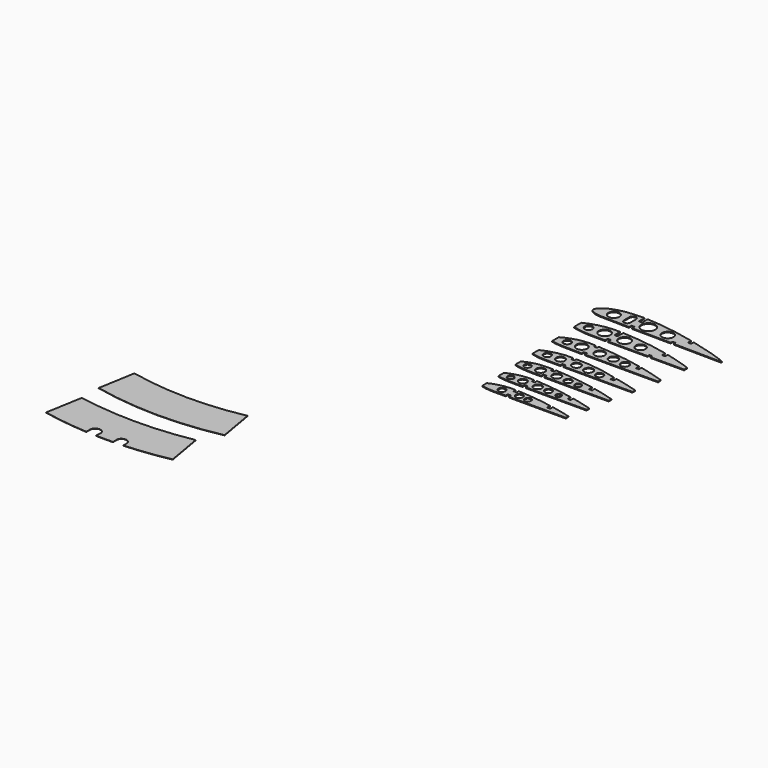
from build123d import *

# Parameters (mm, degrees)
F0_R     = 11.0622151746
F0_R_2   = 13.8024255372
F0_R_3   = 11.3624106866
F1_DEPTH = 1.5875
F0_R_4   = 7.8101063495
F0_R_5   = 11.4767284211
F0_R_6   = 11.8200632114
F0_R_7   = 9.8314713696
F0_R_8   = 7.5345089111
F0_R_9   = 10.9529535392
F0_R_10  = 10.0879453798
F0_R_11  = 8.94065382
F0_R_12  = 8.1637602934
F0_R_13  = 7.4256431867
F0_R_14  = 8.671057932
F0_R_15  = 8.7945693521
F0_R_16  = 8.7340618452
F0_R_17  = 7.4133759763
F0_R_18  = 6.6977708364
F0_R_19  = 8.7178990493
F0_R_20  = 8.6654991063
F0_R_21  = 7.401165003
F0_R_22  = 6.2678513164
F0_R_23  = 6.2709150441
F0_R_24  = 7.8954222452
F0_R_25  = 8.25631298
F0_R_26  = 7.1918059299
F0_R_27  = 5.3987930497
F0_R_28  = 7.1117244514
F0_R_29  = 7.1354689901
F0_R_30  = 6.3367708827
F3_DEPTH = 0.6


# Not quite as in the source:
# - a length typed as a fraction of an inch, garbled in the dataset ("3 / 203.2 mm" for 3/8 in), is restored


with BuildPart() as f1:
    # F0 (on Top) → F1 (new body)
    with BuildSketch(Plane.XY):
        with BuildLine():
            add(Edge.make_bspline(
                [(1167.916059494, 673.0018258095), (1177.8327603734, 680.2652288209), (1199.7700553684, 687.2151988613), (1229.9858664166, 688.5294701263), (1239.9305907432, 688.4111456973)],
                knots=[0, 0, 0, 0, 0.1072430775, 0.1545371155, 0.1545371155, 0.1545371155, 0.1545371155], degree=3))
            add(Edge.make_bspline(
                [(1239.9305907431, 649.5218357149), (1234.8037192798, 649.580005652), (1206.4933945723, 649.9289024866), (1187.615273365, 650.5224661242), (1170.3721430017, 651.1383806137), (1154.5878442427, 659.1619541141), (1162.1400410682, 668.7712303586), (1167.916059494, 673.0018258095)],
                knots=[0.6987548069, 0.6987548069, 0.6987548069, 0.6987548069, 0.7190022786, 0.819021915, 0.8813413001, 0.9375358802, 1, 1, 1, 1], degree=3))
            Line((1239.9305907432, 649.5218357149), (1239.9305907432, 655.275285244))
            Line((1239.9305907432, 655.275285244), (1246.2805907432, 655.275285244))
            Line((1246.2805907432, 655.275285244), (1246.2805907432, 649.4519400523))
            add(Edge.make_bspline(
                [(1324.1934506717, 648.7014399823), (1296.885623439, 648.9761227037), (1268.7687492982, 649.2112810849), (1246.2805907432, 649.4519400523)],
                knots=[0.6063349262, 0.6063349262, 0.6063349262, 0.6063349262, 0.690617928, 0.690617928, 0.690617928, 0.690617928], degree=3))
            Line((1324.1934506717, 648.7014399823), (1324.1934506717, 653.1366514814))
            Line((1324.1934506717, 653.1366514814), (1330.5434506717, 653.1366514814))
            Line((1330.5434506717, 653.1366514814), (1330.5434506717, 648.6366514814))
            add(Edge.make_bspline(
                [(1351.4409561122, 672.2358105918), (1388.7437026108, 663.2075998775), (1443.6632184466, 645.9054628844), (1410.1193627667, 647.6925581204), (1360.1806483068, 648.3297238832), (1330.5434506717, 648.6366514814)],
                knots=[0.3027658347, 0.3027658347, 0.3027658347, 0.3027658347, 0.4360955254, 0.5077565424, 0.5997838404, 0.5997838404, 0.5997838404, 0.5997838404], degree=3))
            Line((1351.4409561122, 672.2358105918), (1351.4409561122, 665.7471058692))
            Line((1351.4409561122, 665.7471058692), (1345.0909561122, 665.7471058692))
            Line((1345.0909561122, 665.7471058692), (1345.0909561122, 673.7471058692))
            add(Edge.make_bspline(
                [(1246.2805907432, 688.2680232189), (1271.1688696042, 687.4499194424), (1304.0430613345, 683.0303025163), (1340.6786828257, 674.7791703585), (1345.0909561122, 673.7471058692)],
                knots=[0.1644584731, 0.1644584731, 0.1644584731, 0.1644584731, 0.2794740967, 0.2952116577, 0.2952116577, 0.2952116577, 0.2952116577], degree=3))
            Line((1246.2805907432, 688.2680232189), (1246.2805907432, 674.230593146))
            Line((1246.2805907432, 674.230593146), (1239.9305907432, 674.230593146))
            Line((1239.9305907432, 674.230593146), (1239.9305907432, 688.4111456973))
        make_face()
        with Locations((1195.444738667, 667.1157416714)):
            Circle(F0_R, mode=Mode.SUBTRACT)
        with BuildLine():
            Line((1219.5305036545, 662.4182462692), (1219.5305036545, 676.5320897102))
            ThreePointArc((1219.5305036545, 676.5320897102), (1221.3903755939, 681.0222177708), (1225.8805036545, 682.8820897102))
            ThreePointArc((1225.8805036545, 682.8820897102), (1230.370631715, 681.0222177708), (1232.2305036545, 676.5320897102))
            Line((1232.2305036545, 676.5320897102), (1232.2305036545, 662.4182462692))
            ThreePointArc((1232.2305036545, 662.4182462692), (1230.370631715, 657.9281182087), (1225.8805036545, 656.0682462692))
            ThreePointArc((1225.8805036545, 656.0682462692), (1221.3903755939, 657.9281182087), (1219.5305036545, 662.4182462692))
        make_face(mode=Mode.SUBTRACT)
        with Locations((1263.8761882742, 667.962765151)):
            Circle(F0_R_2, mode=Mode.SUBTRACT)
        with Locations((1304.3045484236, 666.1560314822)):
            Circle(F0_R_3, mode=Mode.SUBTRACT)
    extrude(amount=F1_DEPTH)


with BuildPart() as f1b:
    # F0 (on Top) → F1, piece 2 (new body)
    with BuildSketch(Plane.XY):
        with BuildLine():
            ThreePointArc((1239.5347647667, 627.8322943831), (1205.0907616018, 625.2747115144), (1172.4393367767, 614.0134930611))
            Line((1172.4393367767, 614.0134930611), (1172.4393367767, 595.8379507065))
            ThreePointArc((1172.4393367767, 595.8379507065), (1188.8403844554, 592.5482978553), (1205.5069208145, 591.1190509796))
            Line((1205.5069208145, 591.1190509796), (1238.8565063656, 590.7864530829))
            Line((1238.8565063656, 590.7864530829), (1238.9804044892, 597.5536530409))
            Line((1238.9804044892, 597.5536530409), (1245.328276646, 597.4374322326))
            Line((1245.328276646, 597.4374322326), (1245.2054009727, 590.7260775566))
            Line((1245.2054009727, 590.7260775566), (1324.0369558334, 590.7260775566))
            Line((1324.0369558334, 590.7260775566), (1324.0369558334, 595.2260775566))
            Line((1324.0369558334, 595.2260775566), (1330.3869558334, 595.2260775566))
            Line((1330.3869558334, 595.2260775566), (1330.3869558334, 590.7260775566))
            Line((1330.3869558334, 590.7260775566), (1397.4435329437, 590.7260775566))
            Line((1397.4435329437, 590.7260775566), (1397.4435329437, 598.5167622566))
            ThreePointArc((1397.4435329437, 598.5167622566), (1372.0702920842, 606.7687201148), (1346.306854179, 613.7071224899))
            Line((1346.306854179, 613.7071224899), (1346.306854179, 607.2013738506))
            Line((1346.306854179, 607.2013738506), (1339.956854179, 607.2013738506))
            Line((1339.956854179, 607.2013738506), (1339.956854179, 615.2013738506))
            ThreePointArc((1339.956854179, 615.2013738506), (1293.0803414498, 623.6815535149), (1245.6241274939, 627.8322943831))
            Line((1245.6241274939, 627.8322943831), (1245.6241274939, 613.596529623))
            Line((1245.6241274939, 613.596529623), (1239.2762553371, 613.7127504313))
            Line((1239.2762553371, 613.7127504313), (1239.5347647667, 627.8322943831))
        make_face()
        with Locations((1192.1851772401, 607.8855288803)):
            Circle(F0_R_4, mode=Mode.SUBTRACT)
        with Locations((1222.5276501158, 609.9544171512)):
            Circle(F0_R_5, mode=Mode.SUBTRACT)
        with Locations((1263.2427941329, 609.4255081453)):
            Circle(F0_R_6, mode=Mode.SUBTRACT)
        with Locations((1297.2076663994, 606.9002884571)):
            Circle(F0_R_7, mode=Mode.SUBTRACT)
    extrude(amount=F1_DEPTH)


with BuildPart() as f1c:
    # F0 (on Top) → F1, piece 3 (new body)
    with BuildSketch(Plane.XY):
        with BuildLine():
            ThreePointArc((1238.4302639777, 567.5054913894), (1205.9071628996, 565.5802991769), (1175.58157444, 553.6715984344))
            Line((1175.58157444, 553.6715984344), (1175.58157444, 537.0760560036))
            ThreePointArc((1175.58157444, 537.0760560036), (1188.6443969552, 534.9011794693), (1201.8571457763, 534.0119727485))
            Line((1201.8571457763, 534.0119727485), (1237.8049937938, 533.3538170941))
            Line((1237.8049937938, 533.3538170941), (1237.9014262066, 538.6208655466))
            Line((1237.9014262066, 538.6208655466), (1244.2492983635, 538.5046447383))
            Line((1244.2492983635, 538.5046447383), (1244.1549937938, 533.3538170941))
            Line((1244.1549937938, 533.3538170941), (1391.0938501358, 533.3538170941))
            Line((1391.0938501358, 533.3538170941), (1391.0938501358, 539.956510067))
            ThreePointArc((1391.0938501358, 539.956510067), (1366.5692128587, 547.2890865784), (1341.7477551274, 553.5436647388))
            Line((1341.7477551274, 553.5436647388), (1341.7477551274, 546.9599847027))
            Line((1341.7477551274, 546.9599847027), (1335.3977551274, 546.9599847027))
            Line((1335.3977551274, 546.9599847027), (1335.3977551274, 554.9599847027))
            ThreePointArc((1335.3977551274, 554.9599847027), (1290.3294142418, 562.9210361512), (1244.7772476653, 567.3407432156))
            Line((1244.7772476653, 567.3407432156), (1244.6992805515, 563.0822521755))
            Line((1244.6992805515, 563.0822521755), (1238.3514083946, 563.1984729838))
            Line((1238.3514083946, 563.1984729838), (1238.4302639777, 567.5054913894))
        make_face()
        with Locations((1196.5373328668, 548.9002638214)):
            Circle(F0_R_8, mode=Mode.SUBTRACT)
        with Locations((1223.6874103546, 551.2469054948)):
            Circle(F0_R_9, mode=Mode.SUBTRACT)
        with Locations((1260.2845484953, 550.3895893185)):
            Circle(F0_R_10, mode=Mode.SUBTRACT)
        with Locations((1288.6651741998, 549.2736514911)):
            Circle(F0_R_11, mode=Mode.SUBTRACT)
        with Locations((1314.2007004166, 546.411754583)):
            Circle(F0_R_12, mode=Mode.SUBTRACT)
    extrude(amount=F1_DEPTH)


with BuildPart() as f1d:
    # F0 (on Top) → F1, piece 4 (new body)
    with BuildSketch(Plane.XY):
        with BuildLine():
            ThreePointArc((1237.4251005242, 512.604401012), (1207.0534787127, 509.9734947859), (1178.2190799713, 500.0773072243))
            Line((1178.2190799713, 500.0773072243), (1178.2190799713, 484.7976267338))
            ThreePointArc((1178.2190799713, 484.7976267338), (1191.7771897913, 481.9047914198), (1205.6064605713, 480.9341690732))
            Line((1205.6064605713, 480.9341690732), (1236.8452621368, 480.9341690732))
            Line((1236.8452621368, 480.9341690732), (1236.94360644, 486.3056431944))
            Line((1236.94360644, 486.3056431944), (1243.2914785969, 486.1894223861))
            Line((1243.2914785969, 486.1894223861), (1243.1952621368, 480.9341690732))
            Line((1243.1952621368, 480.9341690732), (1381.4504146576, 480.9341690732))
            Line((1381.4504146576, 480.9341690732), (1381.4504146576, 487.707555294))
            ThreePointArc((1381.4504146576, 487.707555294), (1358.2067884104, 494.2091325907), (1334.698157452, 499.6754786211))
            Line((1334.698157452, 499.6754786211), (1334.698157452, 493.0386074151))
            Line((1334.698157452, 493.0386074151), (1328.348157452, 493.0386074151))
            Line((1328.348157452, 493.0386074151), (1328.348157452, 501.0386074151))
            ThreePointArc((1328.348157452, 501.0386074151), (1286.4545531704, 509.6444608541), (1243.7698747508, 512.3189741408))
            Line((1243.7698747508, 512.3189741408), (1243.6799109548, 507.4052355091))
            Line((1243.6799109548, 507.4052355091), (1237.3320387979, 507.5214563174))
            Line((1237.3320387979, 507.5214563174), (1237.4251005242, 512.604401012))
        make_face()
        with Locations((1199.2802895632, 495.3084457345)):
            Circle(F0_R_13, mode=Mode.SUBTRACT)
        with Locations((1224.4484491842, 497.0272308374)):
            Circle(F0_R_14, mode=Mode.SUBTRACT)
        with Locations((1256.8231282741, 496.5334318727)):
            Circle(F0_R_15, mode=Mode.SUBTRACT)
        with Locations((1282.3550636385, 495.2315311006)):
            Circle(F0_R_16, mode=Mode.SUBTRACT)
        with Locations((1305.9687719818, 493.0790892843)):
            Circle(F0_R_17, mode=Mode.SUBTRACT)
    extrude(amount=F1_DEPTH)


with BuildPart() as f1e:
    # F0 (on Top) → F1, piece 5 (new body)
    with BuildSketch(Plane.XY):
        with BuildLine():
            ThreePointArc((1226.448059082, 463.0987942219), (1202.7904971813, 460.6432746336), (1180.4225444794, 452.5572061539))
            Line((1180.4225444794, 452.5572061539), (1180.4225444794, 438.625395298))
            ThreePointArc((1180.4225444794, 438.625395298), (1198.2056199078, 435.4494350518), (1216.2387371063, 434.3858659267))
            Line((1216.2387371063, 434.3858659267), (1235.993026729, 434.3858659267))
            Line((1235.993026729, 434.3858659267), (1236.0896060716, 439.6609395487))
            Line((1236.0896060716, 439.6609395487), (1242.4374782285, 439.5447187404))
            Line((1242.4374782285, 439.5447187404), (1242.4374782285, 434.3858659267))
            Line((1242.4374782285, 434.3858659267), (1371.2095022202, 434.3858659267))
            Line((1371.2095022202, 434.3858659267), (1371.3294829039, 440.9390989722))
            ThreePointArc((1371.3294829039, 440.9390989722), (1350.35549391, 446.8344973486), (1329.1513908003, 451.8394896213))
            Line((1329.1513908003, 451.8394896213), (1329.1513908003, 445.1558545853))
            Line((1329.1513908003, 445.1558545853), (1322.8013908003, 445.1558545853))
            Line((1322.8013908003, 445.1558545853), (1322.8013908003, 453.1558545853))
            ThreePointArc((1322.8013908003, 453.1558545853), (1283.0206216553, 459.5382550501), (1242.8632184986, 462.7982552305))
            Line((1242.8632184986, 462.7982552305), (1242.7672873602, 457.558585919))
            Line((1242.7672873602, 457.558585919), (1236.4194152033, 457.6748067273))
            Line((1236.4194152033, 457.6748067273), (1236.5153463417, 462.9144760388))
            Line((1236.5153463417, 462.9144760388), (1226.448059082, 463.0987942219))
        make_face()
        with Locations((1198.0441023861, 447.1582225769)):
            Circle(F0_R_18, mode=Mode.SUBTRACT)
        with Locations((1223.5181704351, 448.3220157835)):
            Circle(F0_R_19, mode=Mode.SUBTRACT)
        with Locations((1255.6049806599, 448.5550950404)):
            Circle(F0_R_20, mode=Mode.SUBTRACT)
        with Locations((1279.9935428, 446.723260048)):
            Circle(F0_R_21, mode=Mode.SUBTRACT)
        with Locations((1301.4470110926, 445.0230332446)):
            Circle(F0_R_22, mode=Mode.SUBTRACT)
    extrude(amount=F1_DEPTH)


with BuildPart() as f1f:
    # F0 (on Top) → F1, piece 6 (new body)
    with BuildSketch(Plane.XY):
        with BuildLine():
            ThreePointArc((1235.6594516904, 416.1663084252), (1209.1630241542, 414.1088185998), (1184.0242147446, 405.4870903492))
            Line((1184.0242147446, 405.4870903492), (1184.0242147446, 391.2636041641))
            ThreePointArc((1184.0242147446, 391.2636041641), (1200.7436711923, 389.2518998835), (1217.5703048706, 388.5799050331))
            Line((1217.5703048706, 388.5799050331), (1235.1543825868, 388.5799050331))
            Line((1235.1543825868, 388.5799050331), (1235.2525718175, 393.9429092365))
            Line((1235.2525718175, 393.9429092365), (1241.6004439743, 393.8266884283))
            Line((1241.6004439743, 393.8266884283), (1241.6004439743, 388.5799050331))
            Line((1241.6004439743, 388.5799050331), (1363.2941246033, 388.5799050331))
            Line((1363.2941246033, 388.5799050331), (1363.2941246033, 395.0207531452))
            ThreePointArc((1363.2941246033, 395.0207531452), (1343.4921381589, 400.4893245671), (1323.4915353344, 405.1797219061))
            Line((1323.4915353344, 405.1797219061), (1323.4915353344, 398.4975746534))
            Line((1323.4915353344, 398.4975746534), (1317.1415353344, 398.4975746534))
            Line((1317.1415353344, 398.4975746534), (1317.1415353344, 406.4975746534))
            ThreePointArc((1317.1415353344, 406.4975746534), (1279.7464885234, 412.6243373089), (1242.0071442111, 416.0402760543))
            Line((1242.0071442111, 416.0402760543), (1241.9052440146, 410.4745823589))
            Line((1241.9052440146, 410.4745823589), (1235.5573718577, 410.5908031672))
            Line((1235.5573718577, 410.5908031672), (1235.6594516904, 416.1663084252))
        make_face()
        with Locations((1202.0222106799, 400.0607971463)):
            Circle(F0_R_23, mode=Mode.SUBTRACT)
        with Locations((1224.8995640209, 401.8878921453)):
            Circle(F0_R_24, mode=Mode.SUBTRACT)
        with Locations((1255.1724300141, 401.5926128944)):
            Circle(F0_R_25, mode=Mode.SUBTRACT)
        with Locations((1276.9705967439, 401.1571388082)):
            Circle(F0_R_26, mode=Mode.SUBTRACT)
        with Locations((1298.9688638208, 399.1346280953)):
            Circle(F0_R_27, mode=Mode.SUBTRACT)
    extrude(amount=F1_DEPTH)


with BuildPart() as f1g:
    # F0 (on Top) → F1, piece 7 (new body)
    with BuildSketch(Plane.XY):
        with BuildLine():
            ThreePointArc((1234.8390406935, 371.3562249229), (1209.2664964888, 369.6497074249), (1184.9279403687, 361.6183996201))
            Line((1184.9279403687, 361.6183996201), (1184.9279403687, 350.1715660095))
            ThreePointArc((1184.9279403687, 350.1715660095), (1196.5799203585, 347.9153883247), (1208.4242105484, 347.1592366695))
            Line((1208.4242105484, 347.1592366695), (1234.3960271193, 347.1592366695))
            Line((1234.3960271193, 347.1592366695), (1234.4912649522, 352.3610382814))
            Line((1234.4912649522, 352.3610382814), (1240.8412649522, 352.3610382814))
            Line((1240.8412649522, 352.3610382814), (1240.8412649522, 347.1592366695))
            Line((1240.8412649522, 347.1592366695), (1354.8233509064, 347.1592366695))
            Line((1354.8233509064, 347.1592366695), (1354.8233509064, 353.4851372242))
            ThreePointArc((1354.8233509064, 353.4851372242), (1335.8224677335, 358.2742529995), (1316.6563549981, 362.3521585743))
            Line((1316.6563549982, 362.3521585743), (1316.6563549982, 355.5396162684))
            Line((1316.6563549982, 355.5396162684), (1310.3063549982, 355.5396162684))
            Line((1310.3063549982, 355.5396162684), (1310.3063549982, 363.5396162684))
            ThreePointArc((1310.3063549982, 363.5396162684), (1275.8769463539, 368.5893998364), (1241.1889477122, 371.3511463703))
            Line((1241.1889477122, 371.3511463703), (1241.0931373904, 366.1180759471))
            Line((1241.0931373904, 366.1180759471), (1234.7452652335, 366.2342967554))
            Line((1234.7452652335, 366.2342967554), (1234.8390406935, 371.3562249229))
        make_face()
        with Locations((1217.8379138224, 358.5398221451)):
            Circle(F0_R_28, mode=Mode.SUBTRACT)
        with Locations((1251.8035414608, 359.3352282035)):
            Circle(F0_R_29, mode=Mode.SUBTRACT)
        with Locations((1270.3444936291, 357.7454706296)):
            Circle(F0_R_30, mode=Mode.SUBTRACT)
    extrude(amount=F1_DEPTH)


with BuildPart() as f3:
    # F2 (on Top) → F3 (new body)
    with BuildSketch(Plane.XY):
        with BuildLine():
            ThreePointArc((960.2080943772, 42.0277000363), (845.8518710306, 31.1486010188), (731.6786653701, 43.8048138309))
            Line((731.6786653701, 43.8048138309), (718.9504504204, -29.9309957772))
            ThreePointArc((718.9504504204, -29.9309957772), (845.887874272, -44.1334078278), (973.01030159, -31.6952988505))
            Line((973.01030159, -31.6952988505), (960.2080943772, 42.0277000363))
        make_face()
    extrude(amount=F3_DEPTH)


with BuildPart() as f3b:
    # F2 (on Top) → F3, piece 2 (new body)
    with BuildSketch(Plane.XY):
        with BuildLine():
            ThreePointArc((948.1315547649, -72.965109332), (833.6791869799, -83.1725668075), (719.2605733871, -72.5934579968))
            Line((719.2605733871, -72.5934579968), (706.4310908318, -146.3117152452))
            ThreePointArc((706.4310908318, -146.3117152452), (751.3147289315, -153.7476115939), (796.6097580808, -158.0130374742))
            Line((796.6097580808, -158.0130374742), (796.6039914502, -148.1126695275))
            ThreePointArc((796.6039914502, -148.1126695275), (806.0978464229, -138.3251010822), (817.1497138002, -146.3117152452))
            Line((817.1497138002, -146.3117152452), (816.30308763, -158.8707447514))
            ThreePointArc((816.30308763, -158.8707447514), (833.6202890611, -159.1292351243), (850.9382085161, -158.924421982))
            Line((850.9382085161, -158.924421982), (850.6739775985, -149.0317221518))
            ThreePointArc((850.6739775985, -149.0317221518), (861.0901640359, -139.8989756074), (870.8099126816, -149.7696638107))
            Line((870.8099126816, -149.7696638107), (870.9612882352, -158.1094499456))
            ThreePointArc((870.9612882352, -158.1094499456), (916.1673052513, -153.9742016225), (960.9724283218, -146.6813832521))
            Line((960.9724283218, -146.6813832521), (948.1315547649, -72.965109332))
        make_face()
    extrude(amount=F3_DEPTH)


solid = Compound([f1.part, f1b.part, f1c.part, f1d.part, f1e.part, f1f.part, f1g.part, f3.part, f3b.part])
